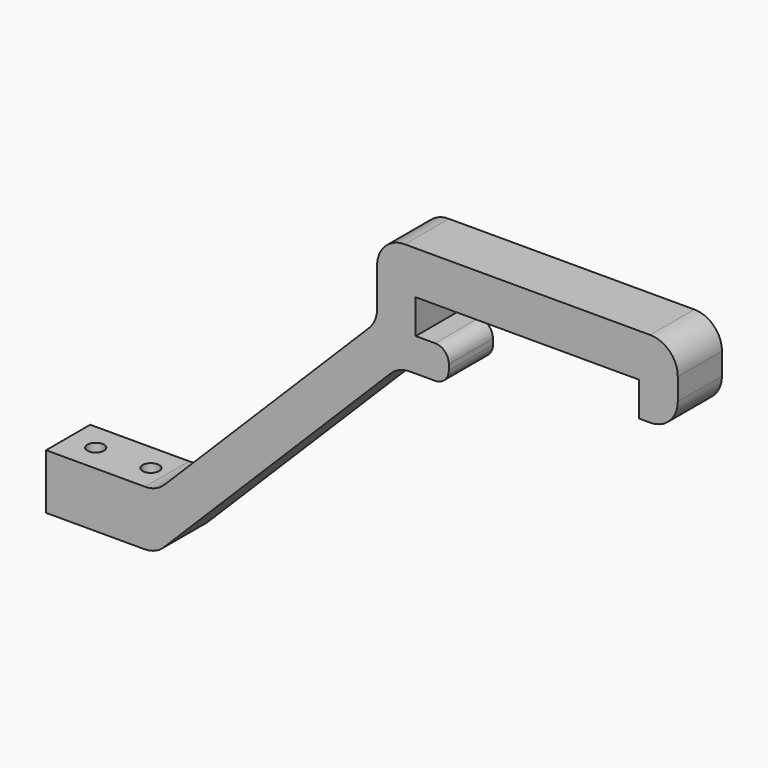
from build123d import *

# Parameters (mm, degrees)
F1_DEPTH = 10
F2_R     = 5
F3_R     = 2.5
F5_R     = 1.5
F6_DEPTH = 25


# Not quite as in the source:
# - two fillets or chamfers of one size are made in one step
# - a feature names something its author has since deleted; it is built from what else it names


with BuildPart() as f1:
    # F0 (on Front) → F1 (new body)
    with BuildSketch(Plane.XZ):
        Polygon((-40.5, 0), (0, 0), (0, -6.2), (7, -6.2), (7, 7.8), (-47.5, 7.8), (-47.5, -6.2), (-87.5, -46.2), (-107.5, -46.2), (-107.5, -56.2), (-87.6005050634, -56.2), (-43.6005050634, -12.2), (-34.5, -12.2), (-34.5, -6.2), (-40.5, -6.2), align=None)
    extrude(amount=F1_DEPTH)

    # F2
    f2_edges = [f1.edges().sort_by_distance(p)[0] for p in [
        (7, -5, -6.2),
        (7, -5, 7.8),
        (-47.5, -5, 7.8),
        (-47.5, -5, -6.2),
        (-87.5, -5, -46.2),
        (-87.600505, -5, -56.2),
        (-43.600505, -5, -12.2),
    ]]
    fillet(f2_edges, radius=F2_R)

    # F3
    f3_edges = [f1.edges().sort_by_distance(p)[0] for p in [
        (-34.5, -5, -12.2),
        (-34.5, -5, -6.2),
    ]]
    fillet(f3_edges, radius=F3_R)

    # F5 (on face) → F6 (cut)
    with BuildSketch(Plane(origin=(0, 0, -56.2), x_dir=(1, 0, 0), z_dir=(0, 0, -1))):
        with Locations((-102.5, 5)):
            Circle(F5_R)
        with Locations((-92.5, 5)):
            Circle(F5_R)
    extrude(amount=-F6_DEPTH, mode=Mode.SUBTRACT)


solid = f1.part
